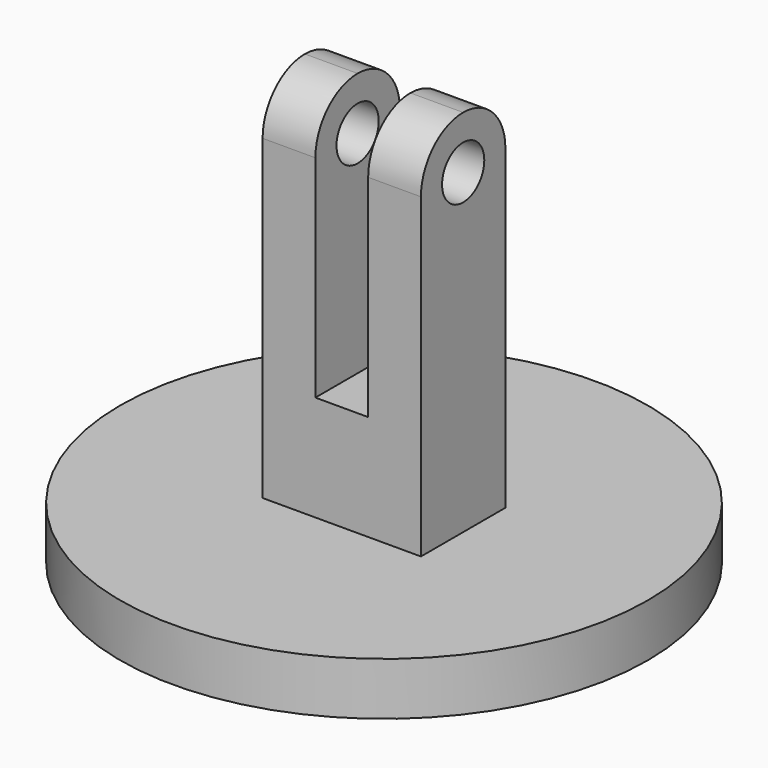
from build123d import *

# Parameters (mm, degrees)
F0_R     = 25
F2_DEPTH = 5
F1_W     = 15
F1_H     = 10
F3_DEPTH = 40
F4_W     = 5
F4_H     = 10
F5_DEPTH = 25
F6_R     = 2.5
F7_DEPTH = 32.501
F8_R     = 4.99999


# Not quite as in the source:
# - a fillet or chamfer is up to 0.001 mm smaller than in the source, because OpenCascade refuses the exact size


with BuildPart() as f2:
    # F0 (on Top) → F2 (new body)
    with BuildSketch(Plane.XY):
        Circle(F0_R)
    extrude(amount=F2_DEPTH)

    # F1 (on Top) → F3 (join)
    with BuildSketch(Plane.XY):
        Rectangle(F1_W, F1_H)
    extrude(amount=F3_DEPTH)

    # F4 (on face) → F5 (cut)
    with BuildSketch(Plane.XY.offset(40)):
        Rectangle(F4_W, F4_H)
    extrude(amount=-F5_DEPTH, mode=Mode.SUBTRACT)

    # F6 (on face) → F7 (cut, through all)
    with BuildSketch(Plane.YZ.offset(7.5)):
        with Locations((0, 35)):
            Circle(F6_R)
    extrude(amount=-F7_DEPTH, mode=Mode.SUBTRACT)

    # F8 (radius 5 in the source; OpenCascade refuses exactly that, so slightly less here)
    f8_edges = [f2.edges().sort_by_distance(p)[0] for p in [
        (-5, 5, 40),
        (-5, -5, 40),
        (5, 5, 40),
        (5, -5, 40),
    ]]
    fillet(f8_edges, radius=F8_R)


solid = f2.part
